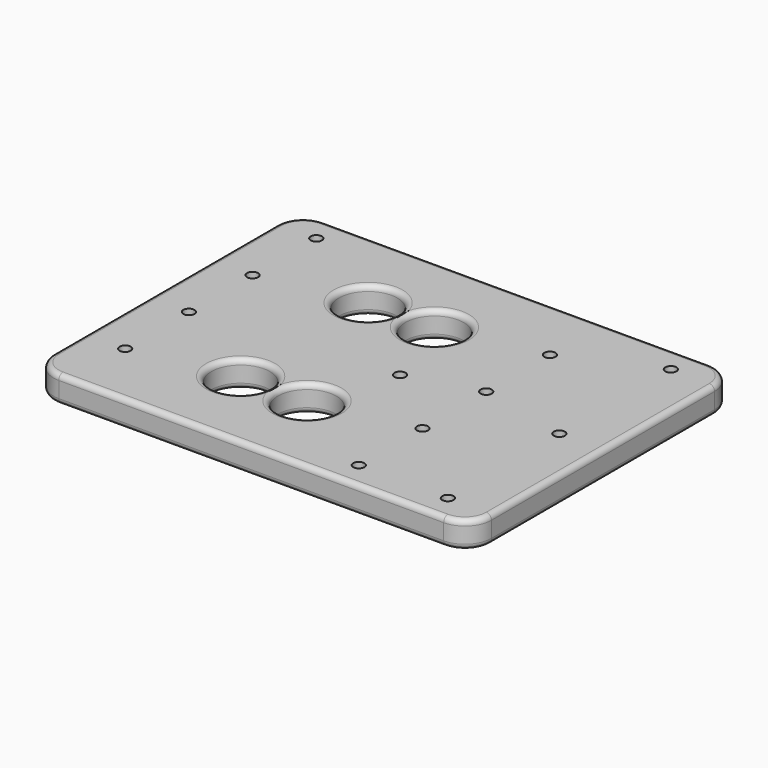
from build123d import *

# Parameters (mm, degrees)
F0_W         = 165
F0_H         = 125
F0_R         = 5.5
F0_R_2       = 11
F0_R_3       = 2.1
F1_DEPTH     = 10
F2_START     = 3
F2_DEPTH     = 7
F3_R         = 10
F4_T1_DEPTH  = 145
F4_T3_DEPTH  = 105
F4_T22_ANGLE = 90
F4_T24_ANGLE = 90
F4_T26_ANGLE = 90
F4_T28_ANGLE = 90
F4_T30_ANGLE = 90
F4_T32_ANGLE = 90
F4_T34_ANGLE = 90
F4_T36_ANGLE = 90


# Not quite as in the source:
# - a fillet or chamfer that OpenCascade refuses, or shapes differently, is made with other operations: its cross-section is extruded or revolved along the edge and cut away or added


with BuildPart() as f1:
    # F0 (on Top) → F1 (new body)
    with BuildSketch(Plane.XY):
        with Locations((82.5, 62.5)):
            Rectangle(F0_W, F0_H)
        with Locations((15, 25)):
            Circle(F0_R, mode=Mode.SUBTRACT)
        with Locations((15, 55)):
            Circle(F0_R, mode=Mode.SUBTRACT)
        with Locations((52.5, 32.5)):
            Circle(F0_R_2, mode=Mode.SUBTRACT)
        with Locations((77.5, 32.5)):
            Circle(F0_R_2, mode=Mode.SUBTRACT)
        with Locations((115, 10)):
            Circle(F0_R, mode=Mode.SUBTRACT)
        with Locations((148.5525276512, 10)):
            Circle(F0_R_3, mode=Mode.SUBTRACT)
        with Locations((115, 40)):
            Circle(F0_R, mode=Mode.SUBTRACT)
        with Locations((15, 85)):
            Circle(F0_R, mode=Mode.SUBTRACT)
        with Locations((52.5, 92.5)):
            Circle(F0_R_2, mode=Mode.SUBTRACT)
        with Locations((77.5, 92.5)):
            Circle(F0_R_2, mode=Mode.SUBTRACT)
        with Locations((15, 115)):
            Circle(F0_R, mode=Mode.SUBTRACT)
        with Locations((88.534809649, 62.5)):
            Circle(F0_R_3, mode=Mode.SUBTRACT)
        with Locations((115, 70)):
            Circle(F0_R, mode=Mode.SUBTRACT)
        with Locations((148.5525276512, 62.5)):
            Circle(F0_R_3, mode=Mode.SUBTRACT)
        with Locations((115, 100)):
            Circle(F0_R, mode=Mode.SUBTRACT)
        with Locations((148.5525276512, 115)):
            Circle(F0_R_3, mode=Mode.SUBTRACT)
    extrude(amount=F1_DEPTH)

    # F0 (on Top) → F2 (join)
    with BuildSketch(Plane.XY.offset(F2_START)):
        with Locations((15, 25)):
            Circle(F0_R)
        with Locations((15, 25)):
            Circle(F0_R_3, mode=Mode.SUBTRACT)
        with Locations((15, 55)):
            Circle(F0_R)
        with Locations((15, 55)):
            Circle(F0_R_3, mode=Mode.SUBTRACT)
        with Locations((115, 10)):
            Circle(F0_R)
        with Locations((115, 10)):
            Circle(F0_R_3, mode=Mode.SUBTRACT)
        with Locations((115, 40)):
            Circle(F0_R)
        with Locations((115, 40)):
            Circle(F0_R_3, mode=Mode.SUBTRACT)
        with Locations((115, 100)):
            Circle(F0_R)
        with Locations((115, 100)):
            Circle(F0_R_3, mode=Mode.SUBTRACT)
        with Locations((115, 70)):
            Circle(F0_R)
        with Locations((115, 70)):
            Circle(F0_R_3, mode=Mode.SUBTRACT)
        with Locations((15, 85)):
            Circle(F0_R)
        with Locations((15, 85)):
            Circle(F0_R_3, mode=Mode.SUBTRACT)
        with Locations((15, 115)):
            Circle(F0_R)
        with Locations((15, 115)):
            Circle(F0_R_3, mode=Mode.SUBTRACT)
    extrude(amount=F2_DEPTH)

    # F3
    f3_edges = [f1.edges().sort_by_distance(p)[0] for p in [
        (165, 0, 5),
        (165, 125, 5),
        (0, 125, 5),
        (0, 0, 5),
    ]]
    fillet(f3_edges, radius=F3_R)

    # F4: fillet of radius 2 on 20 edges, made by hand

    # F4_s2 → F4_t1 (cut)
    with BuildSketch(Plane.YZ.offset(10)):
        with BuildLine():
            ThreePointArc((2, 10), (0.5857864376, 9.4142135624), (0, 8))
            Line((0, 8), (0, 10))
            Line((0, 10), (2, 10))
        make_face()
        with BuildLine():
            ThreePointArc((2, 0), (0.5857864376, 0.5857864376), (0, 2))
            Line((0, 2), (0, 0))
            Line((0, 0), (2, 0))
        make_face()
        with BuildLine():
            ThreePointArc((123, 10), (124.4142135624, 9.4142135624), (125, 8))
            Line((125, 8), (125, 10))
            Line((125, 10), (123, 10))
        make_face()
        with BuildLine():
            ThreePointArc((123, 0), (124.4142135624, 0.5857864376), (125, 2))
            Line((125, 2), (125, 0))
            Line((125, 0), (123, 0))
        make_face()
    extrude(amount=F4_T1_DEPTH, mode=Mode.SUBTRACT)

    # F4_s4 → F4_t3 (cut)
    with BuildSketch(Plane.XZ.offset(-115)):
        with BuildLine():
            ThreePointArc((0, 8), (0.5857864376, 9.4142135624), (2, 10))
            Line((2, 10), (0, 10))
            Line((0, 10), (0, 8))
        make_face()
        with BuildLine():
            ThreePointArc((163, 10), (164.4142135624, 9.4142135624), (165, 8))
            Line((165, 8), (165, 10))
            Line((165, 10), (163, 10))
        make_face()
        with BuildLine():
            ThreePointArc((163, 0), (164.4142135624, 0.5857864376), (165, 2))
            Line((165, 2), (165, 0))
            Line((165, 0), (163, 0))
        make_face()
        with BuildLine():
            ThreePointArc((0, 2), (0.5857864376, 0.5857864376), (2, 0))
            Line((2, 0), (0, 0))
            Line((0, 0), (0, 2))
        make_face()
    extrude(amount=F4_T3_DEPTH, mode=Mode.SUBTRACT)

    # F4_s5 → F4_t6 (revolve, cut)
    with BuildSketch(Plane.XZ.offset(-32.5)):
        with BuildLine():
            ThreePointArc((65.5, 0), (64.0857864376, 0.5857864376), (63.5, 2))
            Line((63.5, 2), (63.5, 0))
            Line((63.5, 0), (65.5, 0))
        make_face()
    revolve(axis=Axis((52.5, 32.5, 0), (0, 0, 1)), mode=Mode.SUBTRACT)

    # F4_s7 → F4_t8 (revolve, cut)
    with BuildSketch(Plane.XZ.offset(-32.5)):
        with BuildLine():
            ThreePointArc((65.5, 10), (64.0857864376, 9.4142135624), (63.5, 8))
            Line((63.5, 8), (63.5, 10))
            Line((63.5, 10), (65.5, 10))
        make_face()
    revolve(axis=Axis((52.5, 32.5, 10), (0, 0, 1)), mode=Mode.SUBTRACT)

    # F4_s9 → F4_t10 (revolve, cut)
    with BuildSketch(Plane.XZ.offset(-32.5)):
        with BuildLine():
            ThreePointArc((90.5, 0), (89.0857864376, 0.5857864376), (88.5, 2))
            Line((88.5, 2), (88.5, 0))
            Line((88.5, 0), (90.5, 0))
        make_face()
    revolve(axis=Axis((77.5, 32.5, 0), (0, 0, 1)), mode=Mode.SUBTRACT)

    # F4_s11 → F4_t12 (revolve, cut)
    with BuildSketch(Plane.XZ.offset(-32.5)):
        with BuildLine():
            ThreePointArc((90.5, 10), (89.0857864376, 9.4142135624), (88.5, 8))
            Line((88.5, 8), (88.5, 10))
            Line((88.5, 10), (90.5, 10))
        make_face()
    revolve(axis=Axis((77.5, 32.5, 10), (0, 0, 1)), mode=Mode.SUBTRACT)

    # F4_s13 → F4_t14 (revolve, cut)
    with BuildSketch(Plane.XZ.offset(-92.5)):
        with BuildLine():
            ThreePointArc((90.5, 0), (89.0857864376, 0.5857864376), (88.5, 2))
            Line((88.5, 2), (88.5, 0))
            Line((88.5, 0), (90.5, 0))
        make_face()
    revolve(axis=Axis((77.5, 92.5, 0), (0, 0, 1)), mode=Mode.SUBTRACT)

    # F4_s15 → F4_t16 (revolve, cut)
    with BuildSketch(Plane.XZ.offset(-92.5)):
        with BuildLine():
            ThreePointArc((90.5, 10), (89.0857864376, 9.4142135624), (88.5, 8))
            Line((88.5, 8), (88.5, 10))
            Line((88.5, 10), (90.5, 10))
        make_face()
    revolve(axis=Axis((77.5, 92.5, 10), (0, 0, 1)), mode=Mode.SUBTRACT)

    # F4_s17 → F4_t18 (revolve, cut)
    with BuildSketch(Plane.XZ.offset(-92.5)):
        with BuildLine():
            ThreePointArc((65.5, 0), (64.0857864376, 0.5857864376), (63.5, 2))
            Line((63.5, 2), (63.5, 0))
            Line((63.5, 0), (65.5, 0))
        make_face()
    revolve(axis=Axis((52.5, 92.5, 0), (0, 0, 1)), mode=Mode.SUBTRACT)

    # F4_s19 → F4_t20 (revolve, cut)
    with BuildSketch(Plane.XZ.offset(-92.5)):
        with BuildLine():
            ThreePointArc((65.5, 10), (64.0857864376, 9.4142135624), (63.5, 8))
            Line((63.5, 8), (63.5, 10))
            Line((63.5, 10), (65.5, 10))
        make_face()
    revolve(axis=Axis((52.5, 92.5, 10), (0, 0, 1)), mode=Mode.SUBTRACT)

    # F4_s21 → F4_t22 (revolve, cut)
    with BuildSketch(Plane.YZ.offset(155)):
        with BuildLine():
            ThreePointArc((123, 0), (124.4142135624, 0.5857864376), (125, 2))
            Line((125, 2), (125, 0))
            Line((125, 0), (123, 0))
        make_face()
    revolve(axis=Axis((155, 115, 0), (0, 0, -1)), revolution_arc=F4_T22_ANGLE, mode=Mode.SUBTRACT)

    # F4_s23 → F4_t24 (revolve, cut)
    with BuildSketch(Plane.XZ.offset(-115)):
        with BuildLine():
            ThreePointArc((2, 0), (0.5857864376, 0.5857864376), (0, 2))
            Line((0, 2), (0, 0))
            Line((0, 0), (2, 0))
        make_face()
    revolve(axis=Axis((10, 115, 0), (0, 0, -1)), revolution_arc=F4_T24_ANGLE, mode=Mode.SUBTRACT)

    # F4_s25 → F4_t26 (revolve, cut)
    with BuildSketch(Plane.XZ.offset(-10)):
        with BuildLine():
            ThreePointArc((2, 0), (0.5857864376, 0.5857864376), (0, 2))
            Line((0, 2), (0, 0))
            Line((0, 0), (2, 0))
        make_face()
    revolve(axis=Axis((10, 10, 0), (0, 0, 1)), revolution_arc=F4_T26_ANGLE, mode=Mode.SUBTRACT)

    # F4_s27 → F4_t28 (revolve, cut)
    with BuildSketch(Plane.YZ.offset(155)):
        with BuildLine():
            ThreePointArc((2, 0), (0.5857864376, 0.5857864376), (0, 2))
            Line((0, 2), (0, 0))
            Line((0, 0), (2, 0))
        make_face()
    revolve(axis=Axis((155, 10, 0), (0, 0, 1)), revolution_arc=F4_T28_ANGLE, mode=Mode.SUBTRACT)

    # F4_s29 → F4_t30 (revolve, cut)
    with BuildSketch(Plane.YZ.offset(155)):
        with BuildLine():
            ThreePointArc((2, 10), (0.5857864376, 9.4142135624), (0, 8))
            Line((0, 8), (0, 10))
            Line((0, 10), (2, 10))
        make_face()
    revolve(axis=Axis((155, 10, 10), (0, 0, 1)), revolution_arc=F4_T30_ANGLE, mode=Mode.SUBTRACT)

    # F4_s31 → F4_t32 (revolve, cut)
    with BuildSketch(Plane.YZ.offset(155)):
        with BuildLine():
            ThreePointArc((123, 10), (124.4142135624, 9.4142135624), (125, 8))
            Line((125, 8), (125, 10))
            Line((125, 10), (123, 10))
        make_face()
    revolve(axis=Axis((155, 115, 10), (0, 0, -1)), revolution_arc=F4_T32_ANGLE, mode=Mode.SUBTRACT)

    # F4_s33 → F4_t34 (revolve, cut)
    with BuildSketch(Plane.XZ.offset(-115)):
        with BuildLine():
            ThreePointArc((0, 8), (0.5857864376, 9.4142135624), (2, 10))
            Line((2, 10), (0, 10))
            Line((0, 10), (0, 8))
        make_face()
    revolve(axis=Axis((10, 115, 10), (0, 0, -1)), revolution_arc=F4_T34_ANGLE, mode=Mode.SUBTRACT)

    # F4_s35 → F4_t36 (revolve, cut)
    with BuildSketch(Plane.XZ.offset(-10)):
        with BuildLine():
            ThreePointArc((0, 8), (0.5857864376, 9.4142135624), (2, 10))
            Line((2, 10), (0, 10))
            Line((0, 10), (0, 8))
        make_face()
    revolve(axis=Axis((10, 10, 10), (0, 0, 1)), revolution_arc=F4_T36_ANGLE, mode=Mode.SUBTRACT)


solid = f1.part
